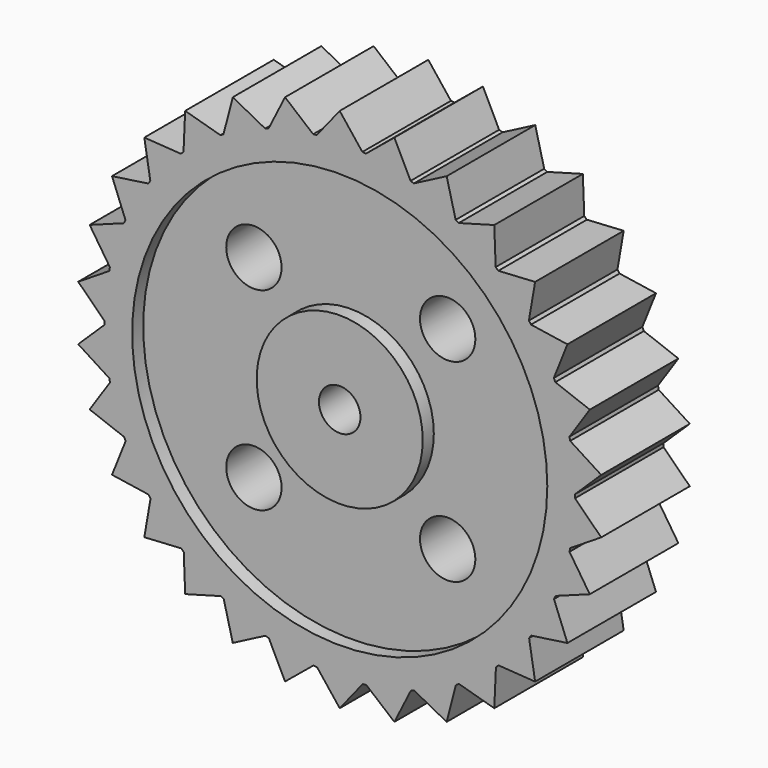
from build123d import *

# Parameters (mm, degrees)
F0_R             = 13.49375
F1_DEPTH         = 3.175
F3_DEPTH         = 6.35
F3_COPIES_COUNT  = 30
F4_R             = 11.90625
F5_DEPTH         = 0.79375
F6_R             = 11.90625
F7_DEPTH         = 0.79375
F9_R             = 4.7625
F10_DEPTH        = 0.79375
F8_R             = 4.7625
F11_DEPTH        = 0.79375
F12_R            = 1.190625
F13_DEPTH        = 6.351
F14_R            = 1.5875
F15_DEPTH        = 5.55725
F15_COPIES_COUNT = 4


# Not quite as in the source:
# - a pattern or mirror of a feature is missing from the dataset's text; its kind, count and spacing are read off the source's solid


with BuildPart() as f1:
    # F0 (on Front) → F1 (new body, symmetric)
    with BuildSketch(Plane.XZ):
        Circle(F0_R)
    extrude(amount=F1_DEPTH, both=True)

    # F2 (on face) → F3 (join, through all)
    with BuildSketch(Plane.XZ.offset(3.175)):
        with BuildLine():
            Line((0, 15.08125), (-1.3182605719, 13.4292024382))
            ThreePointArc((-1.3182605719, 13.4292024382), (-0.6599199427, 13.4776034491), (0, 13.49375))
            Line((0, 13.49375), (0, 15.08125))
        make_face()
        with BuildLine():
            Line((1.2989129689, 13.4310876016), (0, 15.08125))
            Line((0, 15.08125), (0, 13.49375))
            ThreePointArc((0, 13.49375), (0.650211788, 13.4780752963), (1.2989129689, 13.4310876016))
        make_face()
    f3 = extrude(amount=-F3_DEPTH)

    # F3_copies: F3 ×30 about axis
    f3_copies_axis = Axis((0, 0, 0), (0, 1, 0))
    for i in range(1, F3_COPIES_COUNT):
        add(f3.rotate(f3_copies_axis, i * 360 / F3_COPIES_COUNT))

    # F4 (on face) → F5 (cut)
    with BuildSketch(Plane.XZ.offset(3.175)):
        Circle(F4_R)
    extrude(amount=-F5_DEPTH, mode=Mode.SUBTRACT)

    # F6 (on face) → F7 (cut)
    with BuildSketch(Plane(origin=(0, 3.175, 0), x_dir=(-1, 0, 0), z_dir=(0, 1, 0))):
        Circle(F6_R)
    extrude(amount=-F7_DEPTH, mode=Mode.SUBTRACT)

    # F9 (on face) → F10 (join)
    with BuildSketch(Plane(origin=(0, 2.38125, 0), x_dir=(-1, 0, 0), z_dir=(0, 1, 0))):
        Circle(F9_R)
    extrude(amount=F10_DEPTH)

    # F8 (on face) → F11 (join)
    with BuildSketch(Plane.XZ.offset(2.38125)):
        Circle(F8_R)
    extrude(amount=F11_DEPTH)

    # F12 (on face) → F13 (cut, through all)
    with BuildSketch(Plane.XZ.offset(3.175)):
        Circle(F12_R)
    extrude(amount=-F13_DEPTH, mode=Mode.SUBTRACT)

    # F14 (on face) → F15 (cut, through all)
    with BuildSketch(Plane.XZ.offset(2.38125)):
        with Locations((5.55625, -5.55625)):
            Circle(F14_R)
    f15 = extrude(amount=-F15_DEPTH, mode=Mode.SUBTRACT)

    # F15_copies: F15 ×4 about axis
    f15_copies_axis = Axis((0, 0, 0), (0, 1, 0))
    for i in range(1, F15_COPIES_COUNT):
        add(f15.rotate(f15_copies_axis, i * 360 / F15_COPIES_COUNT), mode=Mode.SUBTRACT)


solid = f1.part
